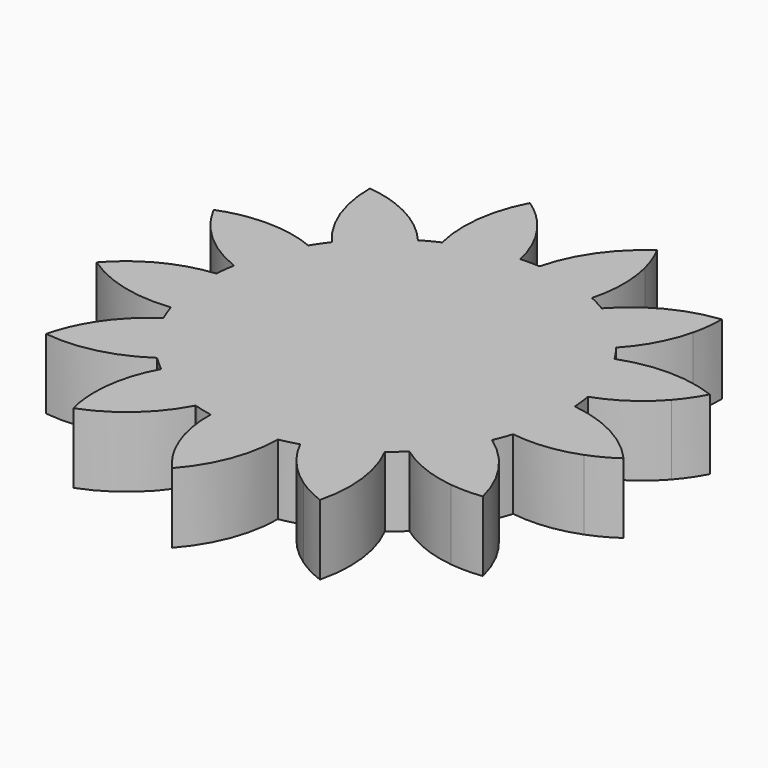
from build123d import *

# Parameters (mm, degrees)
F1_DEPTH = 6.35
F2_COUNT = 13


with BuildPart() as f1:
    # F0 (on Top) → F1 (new body)
    with BuildSketch(Plane.XY):
        with BuildLine():
            ThreePointArc((-2.1437179533, 7.8720496255), (-8.1726662795, 2.7780663468), (-16.0647920269, 2.6720722418))
            ThreePointArc((-16.0647920269, 2.6720722418), (-1.3405858897, -16.2302292777), (16.2855000824, 0))
            ThreePointArc((16.2855000824, 0), (15.6024784663, 4.6669238952), (13.6107061205, 8.9423817764))
            ThreePointArc((13.6107061205, 8.9423817764), (5.9298500897, 5.517014013), (-2.1437179533, 7.8720496255))
        make_face()
        with BuildLine():
            ThreePointArc((-6.7606438886, 14.815910608), (-12.9274256428, 9.9045029751), (-16.0647920269, 2.6720722418))
            ThreePointArc((-16.0647920269, 2.6720722418), (-8.1726662795, 2.7780663468), (-2.1437179533, 7.8720496255))
            ThreePointArc((-2.1437179533, 7.8720496255), (-5.0634420885, 10.9375567243), (-6.7606438886, 14.815910608))
        make_face()
        with BuildLine():
            ThreePointArc((-3.5394354787, 21.5305990191), (-4.554792608, 22.5366665267), (-5.6852551034, 23.4114101898))
            ThreePointArc((-5.6852551034, 23.4114101898), (-7.0109905191, 19.2122527461), (-6.7606438886, 14.815910608))
            ThreePointArc((-6.7606438886, 14.815910608), (-3.8699558436, 15.8190061225), (-0.8426569014, 16.2636847695))
            ThreePointArc((-0.8426569014, 16.2636847695), (-1.8525780021, 19.0704452205), (-3.5394354787, 21.5305990191))
        make_face()
        with BuildLine():
            ThreePointArc((-2.1437179533, 7.8720496255), (5.9298500897, 5.517014013), (13.6107061205, 8.9423817764))
            ThreePointArc((13.6107061205, 8.9423817764), (7.3590855135, 14.5279514502), (-0.8426569014, 16.2636847695))
            ThreePointArc((-0.8426569014, 16.2636847695), (-0.6359958834, 15.0084567204), (-0.5668363347, 13.7382113944))
            ThreePointArc((-0.5668363347, 13.7382113944), (-0.9679319708, 10.7010083415), (-2.1437179533, 7.8720496255))
        make_face()
        with BuildLine():
            ThreePointArc((-0.8426569014, 16.2636847695), (-3.8699558436, 15.8190061225), (-6.7606438886, 14.815910608))
            ThreePointArc((-6.7606438886, 14.815910608), (-5.0634420885, 10.9375567243), (-2.1437179533, 7.8720496255))
            ThreePointArc((-2.1437179533, 7.8720496255), (-0.9679319708, 10.7010083415), (-0.5668363347, 13.7382113944))
            ThreePointArc((-0.5668363347, 13.7382113944), (-0.6359958834, 15.0084567204), (-0.8426569014, 16.2636847695))
        make_face()
    extrude(amount=F1_DEPTH)

    # F2: F1 ×13 about axis
    f2_axis = Axis((0, 0, 6.35), (0, 0, 1))


with BuildPart() as f1_1:
    add(f1.part)
    for i in range(1, F2_COUNT):
        add(f1.part.rotate(f2_axis, i * 360 / F2_COUNT))


solid = f1_1.part
